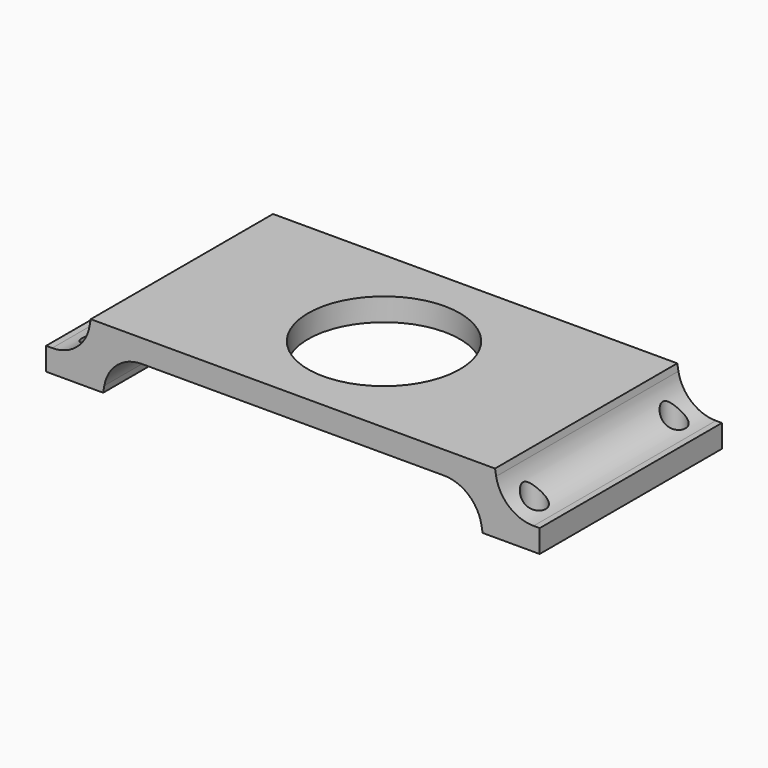
from build123d import *

# Parameters (mm, degrees)
F1_DEPTH = 30
F3_DEPTH = 8.001
F5_D     = 3


with BuildPart() as f1:
    # F0 (on Front) → F1 (new body)
    with BuildSketch(Plane.XZ):
        with BuildLine():
            Line((0, -3), (0, 0))
            Line((0, 0), (-26.6183650965, 0))
            Line((-26.6183650965, 0), (-26.7714593908, -0.8682408883))
            ThreePointArc((-26.7714593908, -0.8682408883), (-28.4815601075, -3.8302222156), (-31.6954981559, -5))
            Line((-31.6954981559, -5), (-32.5, -5))
            Line((-32.5, -5), (-32.5, -8))
            Line((-32.5, -8), (-24.9827011065, -8))
            Line((-24.9827011065, -8), (-24.8296068121, -7.1317591117))
            ThreePointArc((-24.8296068121, -7.1317591117), (-23.1195060955, -4.1697777844), (-19.905568047, -3))
            Line((-19.905568047, -3), (0, -3))
        make_face()
    extrude(amount=F1_DEPTH)

    # F2 (on face) → F3 (cut, through all)
    with BuildSketch(Plane.XY):
        with BuildLine():
            Line((0, -25), (0, -5))
            ThreePointArc((0, -5), (-10, -15), (0, -25))
        make_face()
        with BuildLine():
            ThreePointArc((0, -25), (7.0710678119, -22.0710678119), (10, -15))
            ThreePointArc((10, -15), (7.0710678119, -7.9289321881), (0, -5))
            Line((0, -5), (0, -25))
        make_face()
    extrude(amount=-F3_DEPTH, mode=Mode.SUBTRACT)

    # F5 (through all)
    with Locations(Plane(origin=(0, 0, -8), x_dir=(1, 0, 0), z_dir=(0, 0, -1))):
        with Locations((-29, 26.5), (-29, 3.5)):
            Hole(F5_D / 2)

    # F6: F1 across plane


with BuildPart() as f1_1:
    add(f1.part)
    add(f1.part.mirror(Plane.YZ))


solid = f1_1.part
